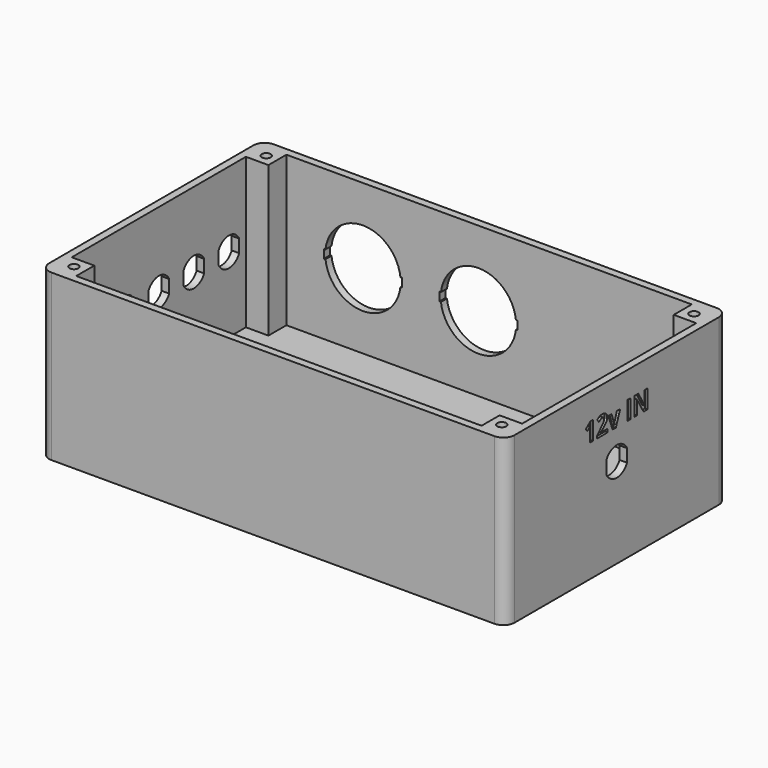
from build123d import *

# Parameters (mm, degrees)
F0_W            = 124
F0_H            = 74
F1_DEPTH        = 44
F2_W            = 120
F2_H            = 70
F3_DEPTH        = 40
F4_W            = 6
F4_H            = 6
F5_DEPTH        = 40
F6_TEXT_SIZE    = 6.9444444444
F7_DEPTH        = 0.7
F9_R            = 5.1
F10_DEPTH       = 1.1
F11_R           = 1.2
F12_DEPTH       = 15
F14_DEPTH       = 2
F16_DEPTH       = 2
F17_R           = 3
F18_DEPTH       = 2
F19_TEXT_SIZE   = 5.5555555556
F19_TEXT_SIZE_2 = 4.1666666667
F20_DEPTH       = 0.75


# Not quite as in the source:
# - Text() gives the source's letters only with a copy of the font that has no kerning and outlines rounded to 1/6400 em; it was checked with that copy


with BuildPart() as f1:
    # F0 (on Top) → F1 (new body)
    with BuildSketch(Plane.XY):
        with Locations((-3.6650604757, -6.3303876668)):
            Rectangle(F0_W, F0_H)
    extrude(amount=F1_DEPTH)

    # F2 (on face) → F3 (cut)
    with BuildSketch(Plane.XY.offset(44)):
        with Locations((-3.6650604757, -6.3303876668)):
            Rectangle(F2_W, F2_H)
    extrude(amount=-F3_DEPTH, mode=Mode.SUBTRACT)

    # F4 (on face) → F5 (join)
    with BuildSketch(Plane.XY.offset(4)):
        with Locations((-60.6650604757, 25.6696123332)):
            Rectangle(F4_W, F4_H)
        with Locations((-60.6650604757, -38.3303876668)):
            Rectangle(F4_W, F4_H)
        with Locations((53.3349395243, -38.3303876668)):
            Rectangle(F4_W, F4_H)
        with Locations((53.3349395243, 25.6696123332)):
            Rectangle(F4_W, F4_H)
    extrude(amount=F5_DEPTH)

    # F6 (on face) → F7 (cut)
    with BuildSketch(Plane.YZ.offset(58.3349395243)):
        with Locations((-17.0573841946, 32.0261743665)):
            Text('12v IN', F6_TEXT_SIZE, font='Open Sans', font_style=FontStyle.BOLD, text_align=(TextAlign.LEFT, TextAlign.BOTTOM))
    extrude(amount=-F7_DEPTH, mode=Mode.SUBTRACT)

    # F9 (on face) → F10 (cut)
    with BuildSketch(Plane(origin=(0, 0, 0), x_dir=(1, 0, 0), z_dir=(0, 0, -1))):
        with Locations((-53.5650604757, 31.2303876668)):
            Circle(F9_R)
        with Locations((-53.5650604757, -18.5696123332)):
            Circle(F9_R)
        with Locations((46.2349395243, -18.5696123332)):
            Circle(F9_R)
        with Locations((46.2349395243, 31.2303876668)):
            Circle(F9_R)
    extrude(amount=-F10_DEPTH, mode=Mode.SUBTRACT)

    # F11 (on face) → F12 (cut)
    with BuildSketch(Plane.XY.offset(44)):
        with Locations((-60.6650604757, -38.3303876668)):
            Circle(F11_R)
        with Locations((53.3349395243, 25.6696123332)):
            Circle(F11_R)
        with Locations((53.3349395243, -38.3303876668)):
            Circle(F11_R)
        with Locations((-60.6650604757, 25.6696123332)):
            Circle(F11_R)
    extrude(amount=-F12_DEPTH, mode=Mode.SUBTRACT)

    # F13 (on face) → F14 (cut, through all)
    with BuildSketch(Plane(origin=(0, 30.6696123332, 0), x_dir=(-1, 0, 0), z_dir=(0, 1, 0))):
        with BuildLine():
            Line((26.8920009996, 22.85), (27.2945435582, 22.85))
            ThreePointArc((27.2945435582, 22.85), (37.2785307377, 13.95), (47.2625179171, 22.85))
            Line((47.2625179171, 22.85), (47.6650604757, 22.85))
            Line((47.6650604757, 22.85), (47.6650604757, 25.15))
            Line((47.6650604757, 25.15), (47.2625179171, 25.15))
            ThreePointArc((47.2625179171, 25.15), (37.2785307377, 34.05), (27.2945435582, 25.15))
            Line((27.2945435582, 25.15), (26.8920009996, 25.15))
            Line((26.8920009996, 25.15), (26.8920009996, 22.85))
        make_face()
        with BuildLine():
            Line((-3.8810584766, 22.85), (-3.478515918, 22.85))
            ThreePointArc((-3.478515918, 22.85), (6.5054712615, 13.95), (16.489458441, 22.85))
            Line((16.489458441, 22.85), (16.8920009996, 22.85))
            Line((16.8920009996, 22.85), (16.8920009996, 25.15))
            Line((16.8920009996, 25.15), (16.489458441, 25.15))
            ThreePointArc((16.489458441, 25.15), (6.5054712615, 34.05), (-3.478515918, 25.15))
            Line((-3.478515918, 25.15), (-3.8810584766, 25.15))
            Line((-3.8810584766, 25.15), (-3.8810584766, 22.85))
        make_face()
    extrude(amount=-F14_DEPTH, mode=Mode.SUBTRACT)

    # F15 (on face) → F16 (cut, through all)
    with BuildSketch(Plane(origin=(-65.6650604757, 0, 0), x_dir=(0, -1, 0), z_dir=(-1, 0, 0))):
        with BuildLine():
            Line((2.8803876668, 25.7088007491), (2.8803876668, 22.2911992509))
            ThreePointArc((2.8803876668, 22.2911992509), (6.3303876668, 20.15), (9.7803876668, 22.2911992509))
            Line((9.7803876668, 22.2911992509), (9.7803876668, 25.7088007491))
            ThreePointArc((9.7803876668, 25.7088007491), (6.3303876668, 27.85), (2.8803876668, 25.7088007491))
        make_face()
        with BuildLine():
            Line((26.1803876668, 25.7329991572), (26.1803876668, 22.3153976591))
            ThreePointArc((26.1803876668, 22.3153976591), (29.6303876668, 20.1741984081), (33.0803876668, 22.3153976591))
            Line((33.0803876668, 22.3153976591), (33.0803876668, 25.7329991572))
            ThreePointArc((33.0803876668, 25.7329991572), (29.6303876668, 27.8741984081), (26.1803876668, 25.7329991572))
        make_face()
        with BuildLine():
            Line((14.5303876668, 25.7088007491), (14.5303876668, 22.2911992509))
            ThreePointArc((14.5303876668, 22.2911992509), (17.9803876668, 20.15), (21.4303876668, 22.2911992509))
            Line((21.4303876668, 22.2911992509), (21.4303876668, 25.7088007491))
            ThreePointArc((21.4303876668, 25.7088007491), (17.9803876668, 27.85), (14.5303876668, 25.7088007491))
        make_face()
        with BuildLine():
            Line((-8.7696123332, 25.7088007491), (-8.7696123332, 22.2911992509))
            ThreePointArc((-8.7696123332, 22.2911992509), (-5.3196123332, 20.15), (-1.8696123332, 22.2911992509))
            Line((-1.8696123332, 22.2911992509), (-1.8696123332, 25.7088007491))
            ThreePointArc((-1.8696123332, 25.7088007491), (-5.3196123332, 27.85), (-8.7696123332, 25.7088007491))
        make_face()
        with BuildLine():
            Line((-13.5496123332, 22.2911992509), (-13.5496123332, 25.7088007491))
            ThreePointArc((-13.5496123332, 25.7088007491), (-16.9996123332, 27.85), (-20.4496123332, 25.7088007491))
            Line((-20.4496123332, 25.7088007491), (-20.4496123332, 22.2911992509))
            ThreePointArc((-20.4496123332, 22.2911992509), (-16.9996123332, 20.15), (-13.5496123332, 22.2911992509))
        make_face()
    extrude(amount=-F16_DEPTH, mode=Mode.SUBTRACT)

    # F17
    f17_edges = [f1.edges().sort_by_distance(p)[0] for p in [
        (-65.66506, -43.330388, 22),
        (58.33494, -43.330388, 22),
        (58.33494, 30.669612, 22),
        (-65.66506, 30.669612, 22),
    ]]
    fillet(f17_edges, radius=F17_R)

    # F8 (on face) → F18 (cut, through all)
    with BuildSketch(Plane.YZ.offset(58.3349395243)):
        with BuildLine():
            Line((-9.7771899819, 25.7088007491), (-9.7771899819, 22.2911992509))
            ThreePointArc((-9.7771899819, 22.2911992509), (-6.3271899819, 20.15), (-2.8771899819, 22.2911992509))
            Line((-2.8771899819, 22.2911992509), (-2.8771899819, 25.7088007491))
            ThreePointArc((-2.8771899819, 25.7088007491), (-6.3271899819, 27.85), (-9.7771899819, 25.7088007491))
        make_face()
    extrude(amount=-F18_DEPTH, mode=Mode.SUBTRACT)

    # F19 (on face) → F20 (cut)
    with BuildSketch(Plane(origin=(-65.6650604757, 0, 0), x_dir=(0, -1, 0), z_dir=(-1, 0, 0))):
        with Locations(Location((-14.9996123332, 32.8585069444), (0, 0, 90))):
            Text('6V', F19_TEXT_SIZE, font='Open Sans', font_style=FontStyle.BOLD, text_align=(TextAlign.LEFT, TextAlign.BOTTOM))
        with Locations(Location((-15.4996123332, 3.685), (0, 0, 90))):
            Text('DRO Z', F19_TEXT_SIZE_2, font='Open Sans', font_style=FontStyle.BOLD, text_align=(TextAlign.LEFT, TextAlign.BOTTOM))
        with Locations(Location((-3.8196123332, 3.685), (0, 0, 90))):
            Text('DRO X', F19_TEXT_SIZE_2, font='Open Sans', font_style=FontStyle.BOLD, text_align=(TextAlign.LEFT, TextAlign.BOTTOM))
        with Locations(Location((-3.3196123332, 32.8585069444), (0, 0, 90))):
            Text('6V', F19_TEXT_SIZE, font='Open Sans', font_style=FontStyle.BOLD, text_align=(TextAlign.LEFT, TextAlign.BOTTOM))
        with Locations(Location((7.8303876668, 2.5), (0, 0, 90))):
            Text('DRO Z2', F19_TEXT_SIZE_2, font='Open Sans', font_style=FontStyle.BOLD, text_align=(TextAlign.LEFT, TextAlign.BOTTOM))
        with Locations(Location((8.3303876668, 32.8585069444), (0, 0, 90))):
            Text('6V', F19_TEXT_SIZE, font='Open Sans', font_style=FontStyle.BOLD, text_align=(TextAlign.LEFT, TextAlign.BOTTOM))
        with Locations(Location((19.4803876668, 2.5), (0, 0, 90))):
            Text('LIGHT 1', F19_TEXT_SIZE_2, font='Open Sans', font_style=FontStyle.BOLD, text_align=(TextAlign.LEFT, TextAlign.BOTTOM))
        with Locations(Location((31.1303876668, 2.5), (0, 0, 90))):
            Text('LIGHT 2', F19_TEXT_SIZE_2, font='Open Sans', font_style=FontStyle.BOLD, text_align=(TextAlign.LEFT, TextAlign.BOTTOM))
        with Locations(Location((19.9803876668, 31.2735069444), (0, 0, 90))):
            Text('12V', F19_TEXT_SIZE, font='Open Sans', font_style=FontStyle.BOLD, text_align=(TextAlign.LEFT, TextAlign.BOTTOM))
        with Locations(Location((31.6303876668, 31.2735069444), (0, 0, 90))):
            Text('12V', F19_TEXT_SIZE, font='Open Sans', font_style=FontStyle.BOLD, text_align=(TextAlign.LEFT, TextAlign.BOTTOM))
    extrude(amount=-F20_DEPTH, mode=Mode.SUBTRACT)


solid = f1.part
